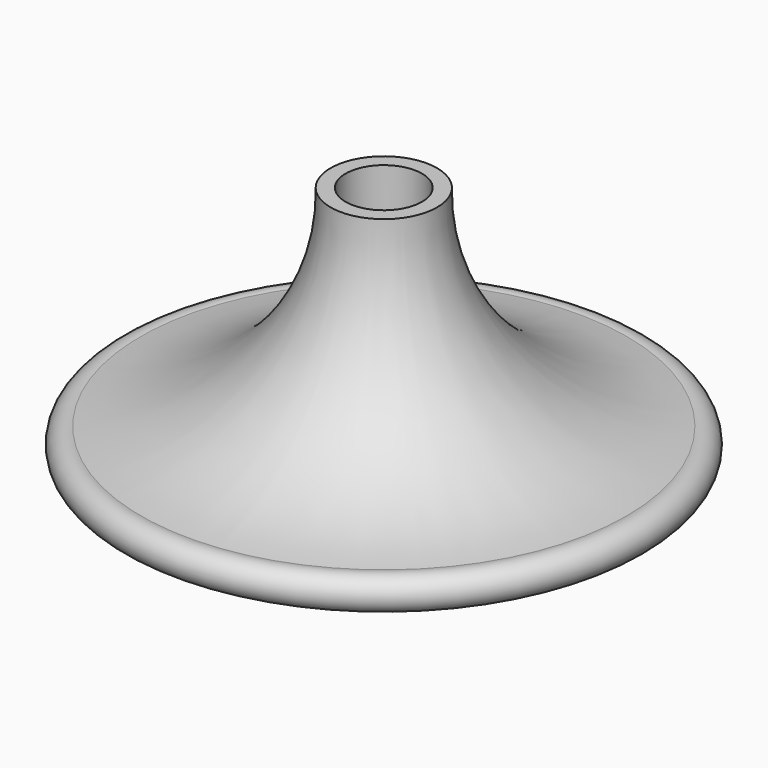
from build123d import *


# Not quite as in the source:
# - a feature names something its author has since deleted; it is built from what else it names


with BuildPart() as f1:
    # F0 (on Front) → F1 (revolve)
    with BuildSketch(Plane.XZ):
        with BuildLine():
            Line((1.579833799, 13.9581533149), (1.579833799, 0))
            Line((1.579833799, 0), (2.8451390099, 0))
            ThreePointArc((2.8451390099, 0), (14.581897199, 8.8414692128), (28.9212949574, 12.0515692979))
            ThreePointArc((28.9212949574, 12.0515692979), (31.4253055765, 13.9538953081), (28.9212949574, 15.8562213182))
            ThreePointArc((28.9212949574, 15.8562213182), (12.6572464777, 23.8517040301), (6.334674079, 40.8361703157))
            Line((6.334674079, 40.8361703157), (4.5473091304, 40.8361703157))
            Line((4.5473091304, 40.8361703157), (4.5473091304, 31.7337363958))
            Line((4.5473091304, 31.7337363958), (0, 31.7337363958))
            Line((0, 31.7337363958), (0, 13.9581533149))
            Line((0, 13.9581533149), (1.579833799, 13.9581533149))
        make_face()
    revolve(axis=Axis((0, 0, 22.8459448554), (0, 0, 1)))


solid = f1.part
